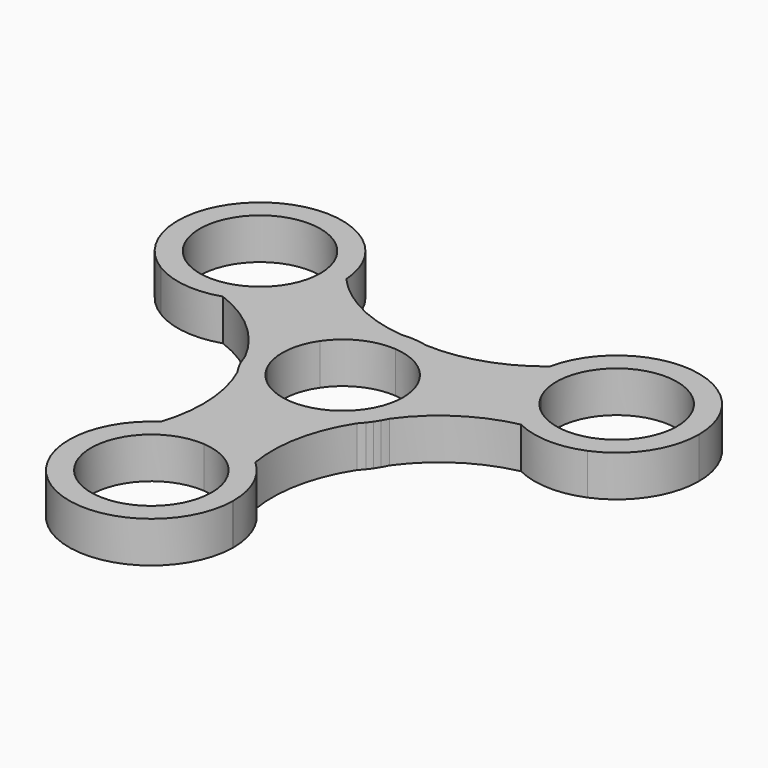
from build123d import *

# Parameters (mm, degrees)
F1_DEPTH = 7.5


with BuildPart() as f1:
    # F0 (on Top) → F1 (new body)
    with BuildSketch(Plane.XY):
        with BuildLine():
            ThreePointArc((9.9070001123, 4.7803084394), (10.7232691199, 2.4518359208), (11, 0))
            ThreePointArc((11, 0), (10.5125414298, -3.2382823666), (9.0933686025, -6.1895595528))
            Line((9.0933686025, -6.1895595528), (12.2828647672, -8.3605456107))
            ThreePointArc((12.2828647672, -8.3605456107), (12.9170786369, -7.3303985813), (13.5985312991, -6.3308724918))
            ThreePointArc((13.5985312991, -6.3308724918), (14.6454424564, -3.2420695947), (15, 0))
            ThreePointArc((15, 0), (14.6226397089, 3.3434126193), (13.5095456076, 6.5186024173))
            Line((13.5095456076, 6.5186024173), (9.9070001123, 4.7803084394))
        make_face()
        with BuildLine():
            ThreePointArc((0.8136315097, 10.9698679922), (6.1895595528, 9.0933686025), (9.9070001123, 4.7803084394))
            Line((9.9070001123, 4.7803084394), (13.5095456076, 6.5186024173))
            ThreePointArc((13.5095456076, 6.5186024173), (9.4154652066, 11.6768580939), (3.5065394099, 14.5843814187))
            ThreePointArc((3.5065394099, 14.5843814187), (2.3000626139, 14.6729470743), (1.0990125047, 14.817545725))
            Line((1.0990125047, 14.817545725), (0.8136315097, 10.9698679922))
        make_face()
        with BuildLine():
            Line((12.2828647672, -8.3605456107), (9.0933686025, -6.1895595528))
            ThreePointArc((9.0933686025, -6.1895595528), (4.7803084394, -9.9070001123), (-0.8136315097, -10.9698679922))
            Line((-0.8136315097, -10.9698679922), (-1.1094975133, -14.9589108985))
            ThreePointArc((-1.1094975133, -14.9589108985), (5.4047231424, -13.9924611043), (10.8771751021, -10.3289429177))
            ThreePointArc((10.8771751021, -10.3289429177), (11.5571136078, -9.3283861911), (12.2828647672, -8.3605456107))
        make_face()
        with BuildLine():
            ThreePointArc((-9.0933686025, 6.1895595528), (-4.7803084394, 9.9070001123), (0.8136315097, 10.9698679922))
            Line((0.8136315097, 10.9698679922), (1.0990125047, 14.817545725))
            ThreePointArc((1.0990125047, 14.817545725), (-0.1102279272, 14.8517175329), (-1.3165692436, 14.9421098051))
            ThreePointArc((-1.3165692436, 14.9421098051), (-7.5897795036, 12.9381315145), (-12.4000480944, 8.4403084812))
            Line((-12.4000480944, 8.4403084812), (-9.0933686025, 6.1895595528))
        make_face()
        with BuildLine():
            Line((22.5159093461, 10.8643373622), (13.5095456076, 6.5186024173))
            ThreePointArc((13.5095456076, 6.5186024173), (14.6226397089, 3.3434126193), (15, 0))
            ThreePointArc((15, 0), (14.6454424564, -3.2420695947), (13.5985312991, -6.3308724918))
            ThreePointArc((13.5985312991, -6.3308724918), (20.5029640043, 0.2861263258), (29.3329113564, 3.958713165))
            ThreePointArc((29.3329113564, 3.958713165), (25.3505772753, 6.8450563796), (22.5159093461, 10.8643373622))
        make_face()
        with BuildLine():
            ThreePointArc((3.5065394099, 14.5843814187), (9.4154652066, 11.6768580939), (13.5095456076, 6.5186024173))
            Line((13.5095456076, 6.5186024173), (22.5159093461, 10.8643373622))
            ThreePointArc((22.5159093461, 10.8643373622), (21.1336653873, 15.5844394293), (21.3524517486, 20.4978999628))
            ThreePointArc((21.3524517486, 20.4978999628), (12.9828009771, 15.8713666716), (3.5065394099, 14.5843814187))
        make_face()
        with BuildLine():
            Line((-1.1094975133, -14.9589108985), (-0.8136315097, -10.9698679922))
            ThreePointArc((-0.8136315097, -10.9698679922), (-6.1895595528, -9.0933686025), (-9.9070001123, -4.7803084394))
            Line((-9.9070001123, -4.7803084394), (-13.381877272, -6.4570001143))
            ThreePointArc((-13.381877272, -6.4570001143), (-12.8068507097, -7.5213189516), (-12.2819620555, -8.6112373133))
            ThreePointArc((-12.2819620555, -8.6112373133), (-7.4098608173, -13.0420076165), (-1.1094975133, -14.9589108985))
        make_face()
        with BuildLine():
            ThreePointArc((12.9903810568, -7.5), (12.6320125035, -7.9264822577), (12.2828647672, -8.3605456107))
            Line((12.2828647672, -8.3605456107), (12.4000480944, -8.4403084812))
            ThreePointArc((12.4000480944, -8.4403084812), (12.7039174324, -7.9756179616), (12.9903810568, -7.5))
        make_face()
        with BuildLine():
            ThreePointArc((13.5985312991, -6.3308724918), (12.9170786369, -7.3303985813), (12.2828647672, -8.3605456107))
            ThreePointArc((12.2828647672, -8.3605456107), (12.6320125035, -7.9264822577), (12.9903810568, -7.5))
            ThreePointArc((12.9903810568, -7.5), (13.3073017494, -6.9221181838), (13.5985312991, -6.3308724918))
        make_face()
        with BuildLine():
            ThreePointArc((11.7417808873, -9.3343763367), (12.0071054891, -8.8445620945), (12.2828647672, -8.3605456107))
            ThreePointArc((12.2828647672, -8.3605456107), (11.5571136078, -9.3283861911), (10.8771751021, -10.3289429177))
            ThreePointArc((10.8771751021, -10.3289429177), (11.3204056104, -9.8411593228), (11.7417808873, -9.3343763367))
        make_face()
        with BuildLine():
            Line((12.4000480944, -8.4403084812), (12.2828647672, -8.3605456107))
            ThreePointArc((12.2828647672, -8.3605456107), (12.0071054891, -8.8445620945), (11.7417808873, -9.3343763367))
            ThreePointArc((11.7417808873, -9.3343763367), (12.0791893759, -8.8934348832), (12.4000480944, -8.4403084812))
        make_face()
        with BuildLine():
            ThreePointArc((-9.9070001123, -4.7803084394), (-10.9698679922, 0.8136315097), (-9.0933686025, 6.1895595528))
            Line((-9.0933686025, 6.1895595528), (-12.4000480944, 8.4403084812))
            ThreePointArc((-12.4000480944, 8.4403084812), (-14.8201883489, 2.3156030104), (-14.383714512, -4.255438501))
            ThreePointArc((-14.383714512, -4.255438501), (-13.8571762217, -5.3445608832), (-13.381877272, -6.4570001143))
            Line((-13.381877272, -6.4570001143), (-9.9070001123, -4.7803084394))
        make_face()
        with BuildLine():
            ThreePointArc((-1.3165692436, 14.9421098051), (-0.1102279272, 14.8517175329), (1.0990125047, 14.817545725))
            ThreePointArc((1.0990125047, 14.817545725), (0.5485287461, 14.9028848578), (0, 15))
            ThreePointArc((0, 15), (-0.6589206796, 14.9855204627), (-1.3165692436, 14.9421098051))
        make_face()
        with BuildLine():
            ThreePointArc((2.2129165924, 14.8358687024), (1.6560627147, 14.8207394268), (1.0990125047, 14.817545725))
            ThreePointArc((1.0990125047, 14.817545725), (2.3000626139, 14.6729470743), (3.5065394099, 14.5843814187))
            ThreePointArc((3.5065394099, 14.5843814187), (2.862491171, 14.7243385011), (2.2129165924, 14.8358687024))
        make_face()
        with BuildLine():
            ThreePointArc((0, 15), (0.5485287461, 14.9028848578), (1.0990125047, 14.817545725))
            Line((1.0990125047, 14.817545725), (1.1094975133, 14.9589108985))
            ThreePointArc((1.1094975133, 14.9589108985), (0.5551290495, 14.9897242049), (0, 15))
        make_face()
        with BuildLine():
            Line((1.1094975133, 14.9589108985), (1.0990125047, 14.817545725))
            ThreePointArc((1.0990125047, 14.817545725), (1.6560627147, 14.8207394268), (2.2129165924, 14.8358687024))
            ThreePointArc((2.2129165924, 14.8358687024), (1.6623458479, 14.9076022982), (1.1094975133, 14.9589108985))
        make_face()
        with BuildLine():
            ThreePointArc((21.3524517486, 20.4978999628), (21.1336653873, 15.5844394293), (22.5159093461, 10.8643373622))
            ThreePointArc((22.5159093461, 10.8643373622), (25.3505772753, 6.8450563796), (29.3329113564, 3.958713165))
            ThreePointArc((29.3329113564, 3.958713165), (35.5965178278, 4.510878729), (41.8094702076, 3.5429554029))
            ThreePointArc((41.8094702076, 3.5429554029), (48.5106507633, 9.0691027835), (51.0254549537, 17.3829397795))
            ThreePointArc((51.0254549537, 17.3829397795), (43.6571032384, 30.2964189566), (28.7910623593, 30.5230906078))
            ThreePointArc((28.7910623593, 30.5230906078), (25.682469555, 25.0573515346), (21.3524517486, 20.4978999628))
        make_face()
        with BuildLine():
            ThreePointArc((47.0254549537, 17.3829397795), (38.4772908745, 6.6596706596), (26.1184548414, 12.6026313401))
            ThreePointArc((26.1184548414, 12.6026313401), (33.5736190329, 28.1062088994), (47.0254549537, 17.3829397795))
        make_face(mode=Mode.SUBTRACT)
        with BuildLine():
            Line((-1.8491625221, -24.9315181641), (-1.1094975133, -14.9589108985))
            ThreePointArc((-1.1094975133, -14.9589108985), (-7.4098608173, -13.0420076165), (-12.2819620555, -8.6112373133))
            ThreePointArc((-12.2819620555, -8.6112373133), (-10.0036893353, -17.8991508435), (-11.238109511, -27.3824029841))
            ThreePointArc((-11.238109511, -27.3824029841), (-6.7472959226, -25.3767721108), (-1.8491625221, -24.9315181641))
        make_face()
        with BuildLine():
            ThreePointArc((10.8771751021, -10.3289429177), (5.4047231424, -13.9924611043), (-1.1094975133, -14.9589108985))
            Line((-1.1094975133, -14.9589108985), (-1.8491625221, -24.9315181641))
            ThreePointArc((-1.8491625221, -24.9315181641), (2.9296877559, -26.0945108152), (7.0754762177, -28.7407156288))
            ThreePointArc((7.0754762177, -28.7407156288), (7.2536062418, -19.1791187943), (10.8771751021, -10.3289429177))
        make_face()
        with BuildLine():
            Line((-20.666746824, 14.0671808019), (-12.4000480944, 8.4403084812))
            ThreePointArc((-12.4000480944, 8.4403084812), (-7.5897795036, 12.9381315145), (-1.3165692436, 14.9421098051))
            ThreePointArc((-1.3165692436, 14.9421098051), (-10.499274669, 17.6130245177), (-18.0948018454, 23.4236898191))
            ThreePointArc((-18.0948018454, 23.4236898191), (-18.073798285, 22.9658035339), (-18.0667949184, 22.5074892831))
            ThreePointArc((-18.0667949184, 22.5074892831), (-18.7315111504, 18.0916496922), (-20.666746824, 14.0671808019))
        make_face()
        with BuildLine():
            ThreePointArc((-14.383714512, -4.255438501), (-14.8201883489, 2.3156030104), (-12.4000480944, 8.4403084812))
            Line((-12.4000480944, 8.4403084812), (-20.666746824, 14.0671808019))
            ThreePointArc((-20.666746824, 14.0671808019), (-24.0633531432, 10.5100713858), (-28.4279279664, 8.242815666))
            ThreePointArc((-28.4279279664, 8.242815666), (-20.236407219, 3.3077521227), (-14.383714512, -4.255438501))
        make_face()
        with BuildLine():
            ThreePointArc((-12.9903810568, -7.5), (-13.1805412496, -6.9764026001), (-13.381877272, -6.4570001143))
            Line((-13.381877272, -6.4570001143), (-13.5095456076, -6.5186024173))
            ThreePointArc((-13.5095456076, -6.5186024173), (-13.2590464819, -7.0141062432), (-12.9903810568, -7.5))
        make_face()
        with BuildLine():
            ThreePointArc((-12.2819620555, -8.6112373133), (-12.8068507097, -7.5213189516), (-13.381877272, -6.4570001143))
            ThreePointArc((-13.381877272, -6.4570001143), (-13.1805412496, -6.9764026001), (-12.9903810568, -7.5))
            ThreePointArc((-12.9903810568, -7.5), (-12.6483810698, -8.0634022789), (-12.2819620555, -8.6112373133))
        make_face()
        with BuildLine():
            ThreePointArc((-13.9546974797, -5.5014923657), (-13.6631682038, -5.9761773322), (-13.381877272, -6.4570001143))
            ThreePointArc((-13.381877272, -6.4570001143), (-13.8571762217, -5.3445608832), (-14.383714512, -4.255438501))
            ThreePointArc((-14.383714512, -4.255438501), (-14.1828967814, -4.8831791784), (-13.9546974797, -5.5014923657))
        make_face()
        with BuildLine():
            Line((-13.5095456076, -6.5186024173), (-13.381877272, -6.4570001143))
            ThreePointArc((-13.381877272, -6.4570001143), (-13.6631682038, -5.9761773322), (-13.9546974797, -5.5014923657))
            ThreePointArc((-13.9546974797, -5.5014923657), (-13.7415352237, -6.014167415), (-13.5095456076, -6.5186024173))
        make_face()
        with BuildLine():
            ThreePointArc((28.7910623593, 30.5230906078), (23.979309946, 26.3210822294), (21.3524517486, 20.4978999628))
            ThreePointArc((21.3524517486, 20.4978999628), (25.682469555, 25.0573515346), (28.7910623593, 30.5230906078))
        make_face()
        with BuildLine():
            ThreePointArc((41.8094702076, 3.5429554029), (35.5965178278, 4.510878729), (29.3329113564, 3.958713165))
            ThreePointArc((29.3329113564, 3.958713165), (35.5258855723, 2.3912610732), (41.8094702076, 3.5429554029))
        make_face()
        with BuildLine():
            ThreePointArc((7.0754762177, -28.7407156288), (2.9296877559, -26.0945108152), (-1.8491625221, -24.9315181641))
            ThreePointArc((-1.8491625221, -24.9315181641), (-6.7472959226, -25.3767721108), (-11.238109511, -27.3824029841))
            ThreePointArc((-11.238109511, -27.3824029841), (-13.8917233412, -33.0829280896), (-17.8364457204, -37.97954102))
            ThreePointArc((-17.8364457204, -37.97954102), (-4.0681575486, -54.849339961), (12.0382406887, -40.195336709))
            ThreePointArc((12.0382406887, -40.195336709), (8.8590682031, -34.7703468338), (7.0754762177, -28.7407156288))
        make_face()
        with BuildLine():
            ThreePointArc((8.0413399646, -39.8904290626), (-11.0193655444, -47.3754158158), (-2.1450285256, -28.9205610704))
            ThreePointArc((-2.1450285256, -28.9205610704), (5.1020454737, -32.4054423093), (8.0413399646, -39.8904290626))
        make_face(mode=Mode.SUBTRACT)
        with BuildLine():
            ThreePointArc((12.0413399646, -39.8904290626), (10.7437493111, -33.7876446078), (7.0754762177, -28.7407156288))
            ThreePointArc((7.0754762177, -28.7407156288), (8.8590682031, -34.7703468338), (12.0382406887, -40.195336709))
            ThreePointArc((12.0382406887, -40.195336709), (12.0405651256, -40.0428907613), (12.0413399646, -39.8904290626))
        make_face()
        with BuildLine():
            ThreePointArc((-28.4279279664, 8.242815666), (-24.0633531432, 10.5100713858), (-20.666746824, 14.0671808019))
            ThreePointArc((-20.666746824, 14.0671808019), (-18.7315111504, 18.0916496922), (-18.0667949184, 22.5074892831))
            ThreePointArc((-18.0667949184, 22.5074892831), (-18.073798285, 22.9658035339), (-18.0948018454, 23.4236898191))
            ThreePointArc((-18.0948018454, 23.4236898191), (-21.7047944866, 28.5720493606), (-23.9730244872, 34.4365856171))
            ThreePointArc((-23.9730244872, 34.4365856171), (-45.4668430127, 30.9477977642), (-40.829303048, 9.6722461012))
            ThreePointArc((-40.829303048, 9.6722461012), (-34.541537758, 9.7129952992), (-28.4279279664, 8.242815666))
        make_face()
        with BuildLine():
            ThreePointArc((-22.0667949184, 22.5074892831), (-22.5542534885, 19.2692069164), (-23.9734263158, 16.3179297302))
            ThreePointArc((-23.9734263158, 16.3179297302), (-43.5793363482, 25.7457716497), (-22.0667949184, 22.5074892831))
        make_face(mode=Mode.SUBTRACT)
        with BuildLine():
            ThreePointArc((-23.9730244872, 34.4365856171), (-21.7047944866, 28.5720493606), (-18.0948018454, 23.4236898191))
            ThreePointArc((-18.0948018454, 23.4236898191), (-19.8338356226, 29.5706888609), (-23.9730244872, 34.4365856171))
        make_face()
        with BuildLine():
            ThreePointArc((-17.8364457204, -37.97954102), (-13.8917233412, -33.0829280896), (-11.238109511, -27.3824029841))
            ThreePointArc((-11.238109511, -27.3824029841), (-15.6920499497, -31.9619499341), (-17.8364457204, -37.97954102))
        make_face()
        with BuildLine():
            ThreePointArc((-40.829303048, 9.6722461012), (-34.7843808387, 7.6061504638), (-28.4279279664, 8.242815666))
            ThreePointArc((-28.4279279664, 8.242815666), (-34.541537758, 9.7129952992), (-40.829303048, 9.6722461012))
        make_face()
    extrude(amount=F1_DEPTH)


solid = f1.part
